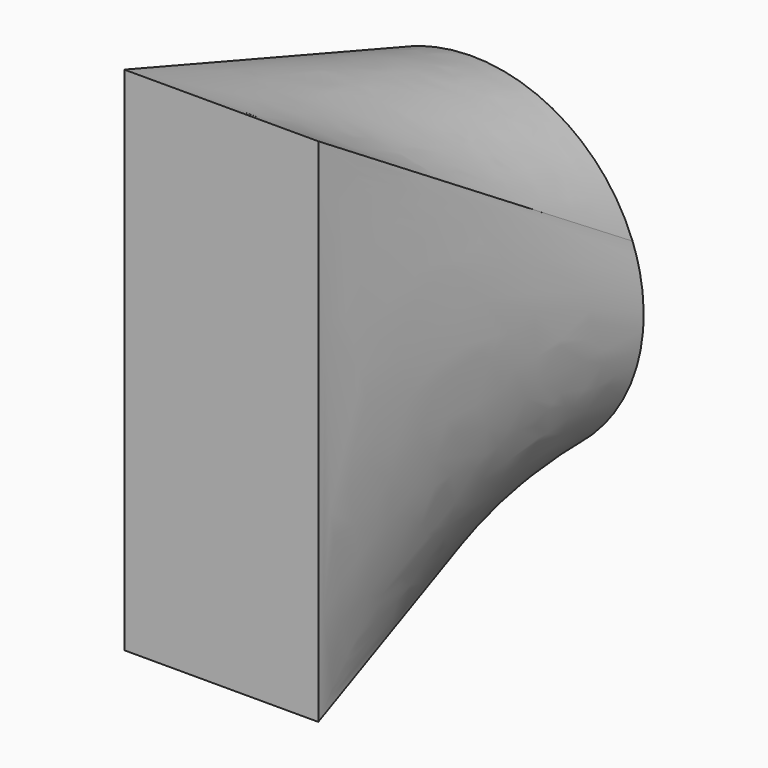
from build123d import *

# Parameters (mm, degrees)
F2_W = 43.3064512908
F2_H = 114.1239330173


# Not quite as in the source:
# - the arcs of a loft's sections are written as splines that run evenly, so that the points pair up as in the source's solid


with BuildPart() as f3:
    # F2 (on offset) → F3 section 0
    with BuildSketch(Plane.XZ.offset(70)):
        Rectangle(F2_W, F2_H)
    # F0 (on Front) → F3 section 1
    with BuildSketch(Plane.XZ):
        with BuildLine():
            add(Edge.make_bspline(
                [(-13.5924092476, 35.8195870657), (-15.9367957389, 34.9299659607), (-18.193506396, 33.8094706474), (-22.4450729848, 31.1496818467), (-24.439823788, 29.6104541278), (-28.0907986632, 26.1723329282), (-29.7469324577, 24.2735244618), (-32.6570107025, 20.1891959329), (-33.9108831954, 18.0037768635), (-35.9682321348, 13.4301994601), (-36.7716577093, 11.0421542169), (-37.8972145774, 6.1550879538), (-38.2193180393, 3.6561877763), (-38.3698283167, -1.3565601307), (-38.1982314106, -3.8702839101), (-37.3679110719, -8.8160763702), (-36.7092081706, -11.2480227564), (-35.8195870657, -13.5924092476)],
                knots=[0, 0, 0, 0, 0.125, 0.125, 0.25, 0.25, 0.375, 0.375, 0.5, 0.5, 0.625, 0.625, 0.75, 0.75, 0.875, 0.875, 1, 1, 1, 1], degree=3))
            add(Edge.make_bspline(
                [(-35.8195870657, -13.5924092476), (-34.9299659607, -15.9367957389), (-33.8094706474, -18.193506396), (-31.1496818467, -22.4450729848), (-29.6104541278, -24.439823788), (-26.1723329282, -28.0907986632), (-24.2735244618, -29.7469324577), (-20.1891959329, -32.6570107025), (-18.0037768635, -33.9108831954), (-13.4301994601, -35.9682321348), (-11.0421542169, -36.7716577093), (-6.1550879538, -37.8972145774), (-3.6561877763, -38.2193180393), (1.3565601307, -38.3698283167), (3.8702839101, -38.1982314106), (8.8160763702, -37.3679110719), (11.2480227564, -36.7092081706), (13.5924092476, -35.8195870657)],
                knots=[0, 0, 0, 0, 0.125, 0.125, 0.25, 0.25, 0.375, 0.375, 0.5, 0.5, 0.625, 0.625, 0.75, 0.75, 0.875, 0.875, 1, 1, 1, 1], degree=3))
            add(Edge.make_bspline(
                [(13.5924092476, -35.8195870657), (15.9367957389, -34.9299659607), (18.193506396, -33.8094706474), (22.4450729848, -31.1496818467), (24.439823788, -29.6104541278), (28.0907986632, -26.1723329282), (29.7469324577, -24.2735244618), (32.6570107025, -20.1891959329), (33.9108831954, -18.0037768635), (35.9682321348, -13.4301994601), (36.7716577093, -11.0421542169), (37.8972145774, -6.1550879538), (38.2193180393, -3.6561877763), (38.3698283167, 1.3565601307), (38.1982314106, 3.8702839101), (37.3679110719, 8.8160763702), (36.7092081706, 11.2480227564), (35.8195870657, 13.5924092476)],
                knots=[0, 0, 0, 0, 0.125, 0.125, 0.25, 0.25, 0.375, 0.375, 0.5, 0.5, 0.625, 0.625, 0.75, 0.75, 0.875, 0.875, 1, 1, 1, 1], degree=3))
            add(Edge.make_bspline(
                [(35.8195870657, 13.5924092476), (34.9299659607, 15.9367957389), (33.8094706474, 18.193506396), (31.1496818467, 22.4450729848), (29.6104541278, 24.439823788), (26.1723329282, 28.0907986632), (24.2735244618, 29.7469324577), (20.1891959329, 32.6570107025), (18.0037768635, 33.9108831954), (13.4301994601, 35.9682321348), (11.0421542169, 36.7716577093), (6.1550879538, 37.8972145774), (3.6561877763, 38.2193180393), (-1.3565601307, 38.3698283167), (-3.8702839101, 38.1982314106), (-8.8160763702, 37.3679110719), (-11.2480227564, 36.7092081706), (-13.5924092476, 35.8195870657)],
                knots=[0, 0, 0, 0, 0.125, 0.125, 0.25, 0.25, 0.375, 0.375, 0.5, 0.5, 0.625, 0.625, 0.75, 0.75, 0.875, 0.875, 1, 1, 1, 1], degree=3))
        make_face()
    loft(ruled=True)


solid = f3.part
